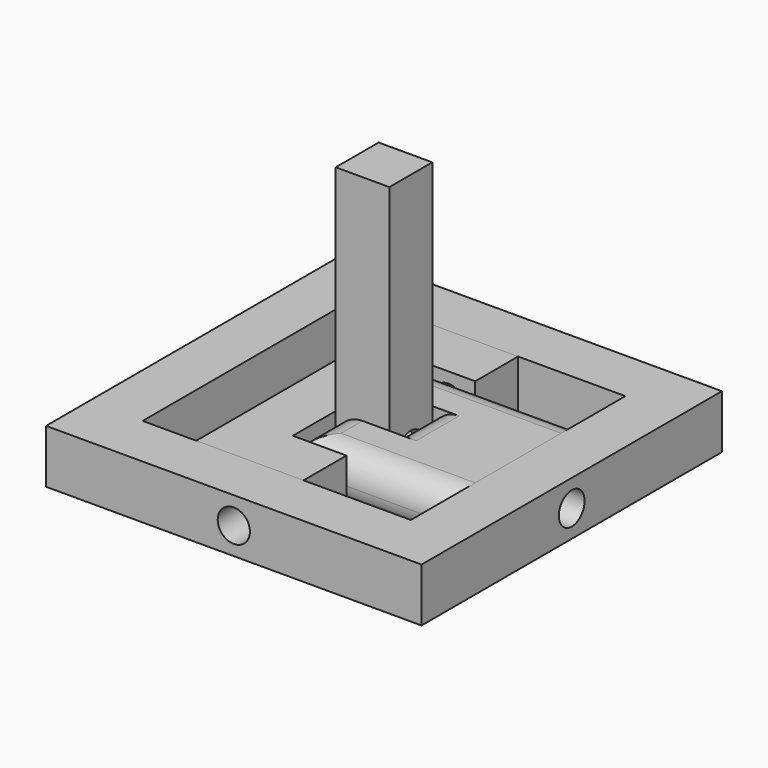
from build123d import *

# Parameters (mm, degrees)
F1_DEPTH       = 5
F2_DEPTH       = 5
F0_W           = 5
F0_H           = 5
F3_DEPTH       = 25
F4_R           = 2.49999
F5_W           = 35
F5_H           = 35
F5_W_2         = 25
F5_H_2         = 25
F6_DEPTH       = 5
F7_R           = 1.5
F8_DEPTH       = 25.001
F9_R           = 1.5
F10_DEPTH      = 30.001
F10_DEPTH_BACK = 5.001


# Not quite as in the source:
# - a fillet or chamfer is up to 0.001 mm smaller than in the source, because OpenCascade refuses the exact size


with BuildPart() as f1:
    # F0 (on Top) → F1 (new body)
    with BuildSketch(Plane.XY):
        Polygon((-2.5, -2.5), (-2.5, 2.5), (-2.5, 7.5), (2.5, 7.5), (2.5, 12.5), (-7.5, 12.5), (-7.5, -12.5), (2.5, -12.5), (2.5, -7.5), (-2.5, -7.5), align=None)
    extrude(amount=F1_DEPTH)


with BuildPart() as f2:
    # F0 (on Top) → F2 (new body)
    with BuildSketch(Plane.XY):
        Polygon((-2.5, 7.5), (-2.5, 2.5), (2.5, 2.5), (2.5, -2.5), (-2.5, -2.5), (-2.5, -7.5), (2.5, -7.5), (12.5, -7.5), (12.5, 7.5), (2.5, 7.5), align=None)
    extrude(amount=F2_DEPTH)

    # F4 (radius 2.5 in the source; OpenCascade refuses exactly that, so slightly less here)
    f4_edges = [f2.edges().sort_by_distance(p)[0] for p in [
        (5, -7.5, 5),
        (5, -7.5, 0),
        (5, 7.5, 5),
        (5, 7.5, 0),
        (2.5, 0, 5),
        (2.5, 0, 0),
        (-2.5, 5, 5),
        (-2.5, 5, 0),
        (-2.5, -5, 0),
        (-2.5, -5, 5),
    ]]
    fillet(f4_edges, radius=F4_R)


with BuildPart() as f3:
    # F0 (on Top) → F3 (new body)
    with BuildSketch(Plane.XY):
        Rectangle(F0_W, F0_H)
    extrude(amount=F3_DEPTH)


with BuildPart() as f6:
    # F5 (on Top) → F6 (new body)
    with BuildSketch(Plane.XY):
        Rectangle(F5_W, F5_H)
        Rectangle(F5_W_2, F5_H_2, mode=Mode.SUBTRACT)
    extrude(amount=F6_DEPTH)


with BuildPart() as f8_tool:
    # F7 (on face) → F8 (new body, through all)
    with BuildSketch(Plane(origin=(-7.5, 0, 0), x_dir=(0, -1, 0), z_dir=(-1, 0, 0))):
        with Locations((0, 2.5)):
            Circle(F7_R)
    extrude(amount=-F8_DEPTH)


with BuildPart() as f1_1:
    add(f1.part)

    # F8: cut by f8_tool
    add(f8_tool.part, mode=Mode.SUBTRACT)


with BuildPart() as f2_1:
    add(f2.part)

    # F8: cut by f8_tool
    add(f8_tool.part, mode=Mode.SUBTRACT)


with BuildPart() as f3_1:
    add(f3.part)

    # F8: cut by f8_tool
    add(f8_tool.part, mode=Mode.SUBTRACT)


with BuildPart() as f6_1:
    add(f6.part)

    # F8: cut by f8_tool
    add(f8_tool.part, mode=Mode.SUBTRACT)


with BuildPart() as f10_tool:
    # F9 (on face) → F10 (new body, two sides)
    with BuildSketch(Plane(origin=(0, 12.5, 0), x_dir=(-1, 0, 0), z_dir=(0, 1, 0))) as f10_sk:
        with Locations((0, 2.5)):
            Circle(F9_R)
    extrude(amount=-F10_DEPTH)
    extrude(f10_sk.sketch, amount=F10_DEPTH_BACK)


with BuildPart() as f1_2:
    add(f1_1.part)

    # F10: cut by f10_tool
    add(f10_tool.part, mode=Mode.SUBTRACT)


with BuildPart() as f2_2:
    add(f2_1.part)

    # F10: cut by f10_tool
    add(f10_tool.part, mode=Mode.SUBTRACT)


with BuildPart() as f3_2:
    add(f3_1.part)

    # F10: cut by f10_tool
    add(f10_tool.part, mode=Mode.SUBTRACT)


with BuildPart() as f6_2:
    add(f6_1.part)

    # F10: cut by f10_tool
    add(f10_tool.part, mode=Mode.SUBTRACT)


solid = Compound([f1_2.part, f2_2.part, f3_2.part, f6_2.part])
